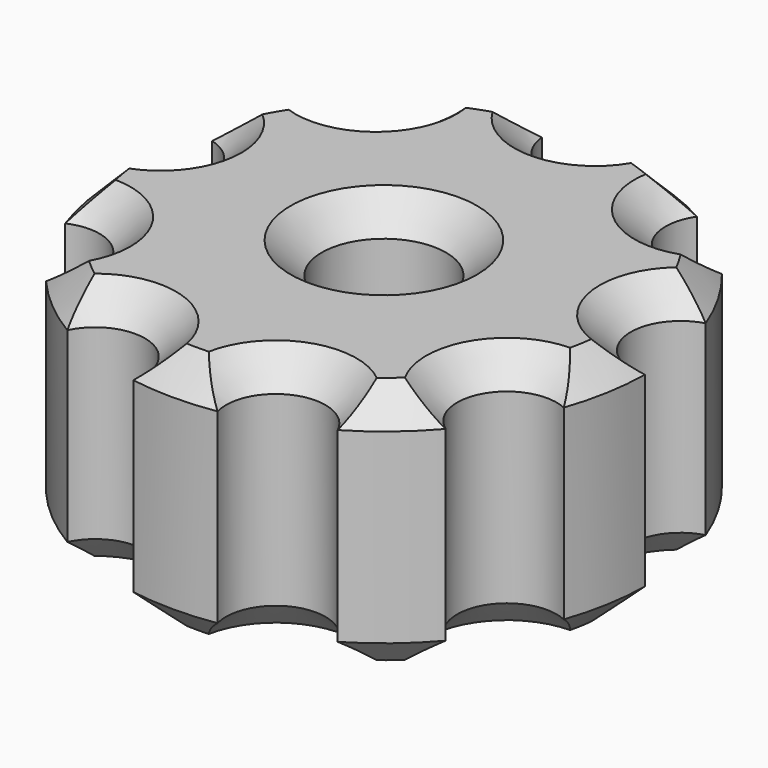
from build123d import *

# Parameters (mm, degrees)
F0_R         = 2
F1_DEPTH     = 8
F2_T2_ANGLE  = 353.6374425132
F2_T4_ANGLE  = 53.075870109
F2_T6_ANGLE  = 353.6374425132
F2_T8_ANGLE  = 53.075870109
F2_T10_ANGLE = 353.6374425132
F2_T12_ANGLE = 53.075870109
F2_T14_ANGLE = 353.6374425132
F2_T16_ANGLE = 53.075870109
F2_T18_ANGLE = 353.6374425132
F2_T20_ANGLE = 53.075870109
F2_T22_ANGLE = 353.6374425132
F2_T24_ANGLE = 53.075870109
F2_T26_ANGLE = 353.6374425132
F2_T28_ANGLE = 53.075870109
F2_T30_ANGLE = 353.6374425132
F2_T32_ANGLE = 53.075870109
F2_T34_ANGLE = 353.6374425132
F2_T36_ANGLE = 53.075870109
F2_T40_ANGLE = 353.6374425132
F2_T42_ANGLE = 53.075870109
F2_T44_ANGLE = 353.6374425132
F2_T46_ANGLE = 53.075870109
F2_T48_ANGLE = 353.6374425132
F2_T50_ANGLE = 53.075870109
F2_T52_ANGLE = 353.6374425132
F2_T54_ANGLE = 53.075870109
F2_T56_ANGLE = 353.6374425132
F2_T58_ANGLE = 53.075870109
F2_T60_ANGLE = 353.6374425132
F2_T62_ANGLE = 53.075870109
F2_T64_ANGLE = 353.6374425132
F2_T66_ANGLE = 53.075870109
F2_T68_ANGLE = 353.6374425132
F2_T70_ANGLE = 53.075870109
F2_T72_ANGLE = 353.6374425132
F2_T74_ANGLE = 53.075870109


# Not quite as in the source:
# - a fillet or chamfer that OpenCascade refuses, or shapes differently, is made with other operations: its cross-section is extruded or revolved along the edge and cut away or added


with BuildPart() as f1:
    # F0 (on Top) → F1 (new body)
    with BuildSketch(Plane.XY):
        with BuildLine():
            ThreePointArc((8.4941564461, -0.1197132759), (6.790249457, 1.197304185), (7.9409517805, 3.0176662871))
            ThreePointArc((7.9409517805, 3.0176662871), (7.3568858051, 4.2475), (6.583851555, 5.3682328285))
            ThreePointArc((6.583851555, 5.3682328285), (4.4320205688, 5.2818764353), (4.1434034849, 7.416011904))
            ThreePointArc((4.1434034849, 7.416011904), (2.9054611176, 7.9826888136), (1.59288935, 8.3443231313))
            ThreePointArc((1.59288935, 8.3443231313), (0, 6.895), (-1.59288935, 8.3443231313))
            ThreePointArc((-1.59288935, 8.3443231313), (-2.9054611176, 7.9826888136), (-4.1434034849, 7.416011904))
            ThreePointArc((-4.1434034849, 7.416011904), (-3.932847998, 6.983297681), (-3.8604807443, 6.5075475443))
            ThreePointArc((-3.8604807443, 6.5075475443), (-4.8429830913, 5.0315066747), (-6.583851555, 5.3682328285))
            ThreePointArc((-6.583851555, 5.3682328285), (-7.3568858051, 4.2475), (-7.9409517805, 3.0176662871))
            ThreePointArc((-7.9409517805, 3.0176662871), (-7.0931527728, 2.4446813329), (-6.7659418618, 1.4751412693))
            ThreePointArc((-6.7659418618, 1.4751412693), (-7.2808481642, 0.2993131919), (-8.4941564461, -0.1197132759))
            ThreePointArc((-8.4941564461, -0.1197132759), (-8.3659418618, -1.4751412693), (-8.022840484, -2.7926789231))
            ThreePointArc((-8.022840484, -2.7926789231), (-6.4924575219, -2.90111085), (-5.7568858051, -4.2475))
            ThreePointArc((-5.7568858051, -4.2475), (-5.9350743771, -4.9812930656), (-6.4299511341, -5.5516442081))
            ThreePointArc((-6.4299511341, -5.5516442081), (-5.4604807443, -6.5075475443), (-4.3507529612, -7.2962986281))
            ThreePointArc((-4.3507529612, -7.2962986281), (-2.5536564486, -6.4218449793), (-1.3054611176, -7.9826888136))
            ThreePointArc((-1.3054611176, -7.9826888136), (-1.318423401, -8.1859405941), (-1.3571002254, -8.3858991157))
            ThreePointArc((-1.3571002254, -8.3858991157), (0, -8.495), (1.3571002254, -8.3858991157))
            ThreePointArc((1.3571002254, -8.3858991157), (2.3582288882, -6.4791806203), (4.3507529612, -7.2962986281))
            ThreePointArc((4.3507529612, -7.2962986281), (5.4604807443, -6.5075475443), (6.4299511341, -5.5516442081))
            ThreePointArc((6.4299511341, -5.5516442081), (5.9712451591, -3.4475), (8.022840484, -2.7926789231))
            ThreePointArc((8.022840484, -2.7926789231), (8.3659418618, -1.4751412693), (8.4941564461, -0.1197132759))
        make_face()
        Circle(F0_R, mode=Mode.SUBTRACT)
    extrude(amount=F1_DEPTH)

    # F2: chamfer of 1 on 38 edges, made by hand

    # F2_s1 → F2_t2 (revolve, cut)
    with BuildSketch(Plane(origin=(0.2580100634, 0.3945620225, 0), x_dir=(0, 0, 1), z_dir=(0.5472897836, 0.8369431837, 0))):
        Polygon((7, 10.0819087839), (8, 11.0819087839), (8, 10.0819087839), align=None)
    revolve(axis=Axis((7.3568858051, -4.2475, 8), (0, 0, -1)), revolution_arc=F2_T2_ANGLE, mode=Mode.SUBTRACT)

    # F2_s3 → F2_t4 (revolve, cut)
    with BuildSketch(Plane(origin=(0, 0, 0), x_dir=(0, 0, 1), z_dir=(-0.5953548832, -0.8034628573, 0))):
        Polygon((8, -7.495), (7, -8.495), (8, -8.495), align=None)
    revolve(axis=Axis((0, 0, 8), (0, 0, 1)), revolution_arc=F2_T4_ANGLE, mode=Mode.SUBTRACT)

    # F2_s5 → F2_t6 (revolve, cut)
    with BuildSketch(Plane(origin=(-0.055972404, 0.4680977167, 0), x_dir=(0, 0, 1), z_dir=(-0.118728411, 0.9929267669, 0))):
        Polygon((8, 11.0819087839), (7, 10.0819087839), (8, 10.0819087839), align=None)
    revolve(axis=Axis((8.3659418618, 1.4751412693, 8), (0, 0, -1)), revolution_arc=F2_T6_ANGLE, mode=Mode.SUBTRACT)

    # F2_s7 → F2_t8 (revolve, cut)
    with BuildSketch(Plane(origin=(0, 0, 0), x_dir=(0, 0, 1), z_dir=(0.0603876695, -0.9981749994, 0))):
        Polygon((8, -7.495), (7, -8.495), (8, -8.495), align=None)
    revolve(axis=Axis((0, 0, 8), (0, 0, 1)), revolution_arc=F2_T8_ANGLE, mode=Mode.SUBTRACT)

    # F2_s9 → F2_t10 (revolve, cut)
    with BuildSketch(Plane(origin=(-0.3437647615, 0.322605287, 0), x_dir=(0, 0, 1), z_dir=(-0.7291922626, 0.6843088807, 0))):
        Polygon((8, 11.0819087839), (7, 10.0819087839), (8, 10.0819087839), align=None)
    revolve(axis=Axis((5.4604807443, 6.5075475443, 8), (0, 0, -1)), revolution_arc=F2_T10_ANGLE, mode=Mode.SUBTRACT)

    # F2_s11 → F2_t12 (revolve, cut)
    with BuildSketch(Plane(origin=(0, 0, 0), x_dir=(0, 0, 1), z_dir=(0.6878741606, -0.7258299658, 0))):
        Polygon((8, -7.495), (7, -8.495), (8, -8.495), align=None)
    revolve(axis=Axis((0, 0, 8), (0, 0, 1)), revolution_arc=F2_T12_ANGLE, mode=Mode.SUBTRACT)

    # F2_s13 → F2_t14 (revolve, cut)
    with BuildSketch(Plane(origin=(-0.4707057666, 0.0261622581, 0), x_dir=(0, 0, 1), z_dir=(-0.9984589504, 0.0554952639, 0))):
        Polygon((8, 11.0819087839), (7, 10.0819087839), (8, 10.0819087839), align=None)
    revolve(axis=Axis((0, 8.495, 8), (0, 0, -1)), revolution_arc=F2_T14_ANGLE, mode=Mode.SUBTRACT)

    # F2_s15 → F2_t16 (revolve, cut)
    with BuildSketch(Plane(origin=(0, 0, 0), x_dir=(0, 0, 1), z_dir=(0.993496687, -0.1138610245, 0))):
        Polygon((8, -7.495), (7, -8.495), (8, -8.495), align=None)
    revolve(axis=Axis((0, 0, 8), (0, 0, 1)), revolution_arc=F2_T16_ANGLE, mode=Mode.SUBTRACT)

    # F2_s17 → F2_t18 (revolve, cut)
    with BuildSketch(Plane(origin=(0.3437647615, 0.322605287, 0), x_dir=(0, 0, 1), z_dir=(0.7291922626, 0.6843088807, 0))):
        Polygon((8, -11.0819087839), (7, -10.0819087839), (8, -10.0819087839), align=None)
    revolve(axis=Axis((-5.4604807443, 6.5075475443, 8), (0, 0, 1)), revolution_arc=F2_T18_ANGLE, mode=Mode.SUBTRACT)

    # F2_s19 → F2_t20 (revolve, cut)
    with BuildSketch(Plane(origin=(0, 0, 0), x_dir=(0, 0, 1), z_dir=(0.8342510721, 0.5513847556, 0))):
        Polygon((8, -7.495), (7, -8.495), (8, -8.495), align=None)
    revolve(axis=Axis((0, 0, 8), (0, 0, 1)), revolution_arc=F2_T20_ANGLE, mode=Mode.SUBTRACT)

    # F2_s21 → F2_t22 (revolve, cut)
    with BuildSketch(Plane(origin=(0.055972404, 0.4680977167, 0), x_dir=(0, 0, 1), z_dir=(0.118728411, 0.9929267669, 0))):
        Polygon((8, -11.0819087839), (7, -10.0819087839), (8, -10.0819087839), align=None)
    revolve(axis=Axis((-8.3659418618, 1.4751412693, 8), (0, 0, 1)), revolution_arc=F2_T22_ANGLE, mode=Mode.SUBTRACT)

    # F2_s23 → F2_t24 (revolve, cut)
    with BuildSketch(Plane(origin=(0, 0, 0), x_dir=(0, 0, 1), z_dir=(0.2846501089, 0.9586314806, 0))):
        Polygon((8, -7.495), (7, -8.495), (8, -8.495), align=None)
    revolve(axis=Axis((0, 0, 8), (0, 0, 1)), revolution_arc=F2_T24_ANGLE, mode=Mode.SUBTRACT)

    # F2_s25 → F2_t26 (revolve, cut)
    with BuildSketch(Plane(origin=(-0.2580100634, 0.3945620225, 0), x_dir=(0, 0, 1), z_dir=(-0.5472897836, 0.8369431837, 0))):
        Polygon((8, -11.0819087839), (7, -10.0819087839), (8, -10.0819087839), align=None)
    revolve(axis=Axis((-7.3568858051, -4.2475, 8), (0, 0, 1)), revolution_arc=F2_T26_ANGLE, mode=Mode.SUBTRACT)

    # F2_s27 → F2_t28 (revolve, cut)
    with BuildSketch(Plane(origin=(0, 0, 0), x_dir=(0, 0, 1), z_dir=(-0.3981418038, 0.9173238818, 0))):
        Polygon((8, -7.495), (7, -8.495), (8, -8.495), align=None)
    revolve(axis=Axis((0, 0, 8), (0, 0, 1)), revolution_arc=F2_T28_ANGLE, mode=Mode.SUBTRACT)

    # F2_s29 → F2_t30 (revolve, cut)
    with BuildSketch(Plane(origin=(-0.4512667547, 0.1364063729, 0), x_dir=(0, 0, 1), z_dir=(-0.957225006, 0.2893445833, 0))):
        Polygon((8, -11.0819087839), (7, -10.0819087839), (8, -10.0819087839), align=None)
    revolve(axis=Axis((-2.9054611176, -7.9826888136, 8), (0, 0, 1)), revolution_arc=F2_T30_ANGLE, mode=Mode.SUBTRACT)

    # F2_s31 → F2_t32 (revolve, cut)
    with BuildSketch(Plane(origin=(0, 0, 0), x_dir=(0, 0, 1), z_dir=(-0.8946387416, 0.4467902438, 0))):
        Polygon((8, -7.495), (7, -8.495), (8, -8.495), align=None)
    revolve(axis=Axis((0, 0, 8), (0, 0, 1)), revolution_arc=F2_T32_ANGLE, mode=Mode.SUBTRACT)

    # F2_s33 → F2_t34 (revolve, cut)
    with BuildSketch(Plane(origin=(0.4512667547, 0.1364063729, 0), x_dir=(0, 0, 1), z_dir=(0.957225006, 0.2893445833, 0))):
        Polygon((8, 11.0819087839), (7, 10.0819087839), (8, 10.0819087839), align=None)
    revolve(axis=Axis((2.9054611176, -7.9826888136, 8), (0, 0, -1)), revolution_arc=F2_T34_ANGLE, mode=Mode.SUBTRACT)

    # F2_s35 → F2_t36 (revolve, cut)
    with BuildSketch(Plane(origin=(0, 0, 0), x_dir=(0, 0, 1), z_dir=(-0.9725242695, -0.2328015148, 0))):
        Polygon((8, -7.495), (7, -8.495), (8, -8.495), align=None)
    revolve(axis=Axis((0, 0, 8), (0, 0, 1)), revolution_arc=F2_T36_ANGLE, mode=Mode.SUBTRACT)

    # F2_s37 → F2_t38 (revolve, cut)
    with BuildSketch(Plane.XZ):
        Polygon((3, 8), (2, 7), (2, 8), align=None)
    revolve(axis=Axis((0, 0, 8), (0, 0, 1)), mode=Mode.SUBTRACT)

    # F2_s39 → F2_t40 (revolve, cut)
    with BuildSketch(Plane(origin=(0.2580100634, 0.3945620225, 0), x_dir=(0, 0, 1), z_dir=(0.5472897836, 0.8369431837, 0))):
        Polygon((1, 10.0819087839), (0, 11.0819087839), (0, 10.0819087839), align=None)
    revolve(axis=Axis((7.3568858051, -4.2475, 0), (0, 0, -1)), revolution_arc=F2_T40_ANGLE, mode=Mode.SUBTRACT)

    # F2_s41 → F2_t42 (revolve, cut)
    with BuildSketch(Plane(origin=(0, 0, 0), x_dir=(0, 0, 1), z_dir=(-0.5953548832, -0.8034628573, 0))):
        Polygon((0, -7.495), (1, -8.495), (0, -8.495), align=None)
    revolve(axis=Axis((0, 0, 0), (0, 0, 1)), revolution_arc=F2_T42_ANGLE, mode=Mode.SUBTRACT)

    # F2_s43 → F2_t44 (revolve, cut)
    with BuildSketch(Plane(origin=(-0.055972404, 0.4680977167, 0), x_dir=(0, 0, 1), z_dir=(-0.118728411, 0.9929267669, 0))):
        Polygon((1, 10.0819087839), (0, 11.0819087839), (0, 10.0819087839), align=None)
    revolve(axis=Axis((8.3659418618, 1.4751412693, 0), (0, 0, -1)), revolution_arc=F2_T44_ANGLE, mode=Mode.SUBTRACT)

    # F2_s45 → F2_t46 (revolve, cut)
    with BuildSketch(Plane(origin=(0, 0, 0), x_dir=(0, 0, 1), z_dir=(0.0603876695, -0.9981749994, 0))):
        Polygon((1, -8.495), (0, -7.495), (0, -8.495), align=None)
    revolve(axis=Axis((0, 0, 0), (0, 0, 1)), revolution_arc=F2_T46_ANGLE, mode=Mode.SUBTRACT)

    # F2_s47 → F2_t48 (revolve, cut)
    with BuildSketch(Plane(origin=(-0.3437647615, 0.322605287, 0), x_dir=(0, 0, 1), z_dir=(-0.7291922626, 0.6843088807, 0))):
        Polygon((1, 10.0819087839), (0, 11.0819087839), (0, 10.0819087839), align=None)
    revolve(axis=Axis((5.4604807443, 6.5075475443, 0), (0, 0, -1)), revolution_arc=F2_T48_ANGLE, mode=Mode.SUBTRACT)

    # F2_s49 → F2_t50 (revolve, cut)
    with BuildSketch(Plane(origin=(0, 0, 0), x_dir=(0, 0, 1), z_dir=(0.6878741606, -0.7258299658, 0))):
        Polygon((1, -8.495), (0, -7.495), (0, -8.495), align=None)
    revolve(axis=Axis((0, 0, 0), (0, 0, 1)), revolution_arc=F2_T50_ANGLE, mode=Mode.SUBTRACT)

    # F2_s51 → F2_t52 (revolve, cut)
    with BuildSketch(Plane(origin=(-0.4707057666, 0.0261622581, 0), x_dir=(0, 0, 1), z_dir=(-0.9984589504, 0.0554952639, 0))):
        Polygon((1, 10.0819087839), (0, 11.0819087839), (0, 10.0819087839), align=None)
    revolve(axis=Axis((0, 8.495, 0), (0, 0, -1)), revolution_arc=F2_T52_ANGLE, mode=Mode.SUBTRACT)

    # F2_s53 → F2_t54 (revolve, cut)
    with BuildSketch(Plane(origin=(0, 0, 0), x_dir=(0, 0, 1), z_dir=(0.993496687, -0.1138610245, 0))):
        Polygon((1, -8.495), (0, -7.495), (0, -8.495), align=None)
    revolve(axis=Axis((0, 0, 0), (0, 0, 1)), revolution_arc=F2_T54_ANGLE, mode=Mode.SUBTRACT)

    # F2_s55 → F2_t56 (revolve, cut)
    with BuildSketch(Plane(origin=(-0.3773983122, -0.2825223821, 0), x_dir=(0, 0, 1), z_dir=(-0.8005355987, -0.5992852036, 0))):
        Polygon((1, 10.0819087839), (0, 11.0819087839), (0, 10.0819087839), align=None)
    revolve(axis=Axis((-5.4604807443, 6.5075475443, 0), (0, 0, -1)), revolution_arc=F2_T56_ANGLE, mode=Mode.SUBTRACT)

    # F2_s57 → F2_t58 (revolve, cut)
    with BuildSketch(Plane(origin=(0, 0, 0), x_dir=(0, 0, 1), z_dir=(0.8342510721, 0.5513847556, 0))):
        Polygon((1, -8.495), (0, -7.495), (0, -8.495), align=None)
    revolve(axis=Axis((0, 0, 0), (0, 0, 1)), revolution_arc=F2_T58_ANGLE, mode=Mode.SUBTRACT)

    # F2_s59 → F2_t60 (revolve, cut)
    with BuildSketch(Plane(origin=(-0.1075019932, -0.4590116599, 0), x_dir=(0, 0, 1), z_dir=(-0.2280327434, -0.973653464, 0))):
        Polygon((1, 10.0819087839), (0, 11.0819087839), (0, 10.0819087839), align=None)
    revolve(axis=Axis((-8.3659418618, 1.4751412693, 0), (0, 0, -1)), revolution_arc=F2_T60_ANGLE, mode=Mode.SUBTRACT)

    # F2_s61 → F2_t62 (revolve, cut)
    with BuildSketch(Plane(origin=(0, 0, 0), x_dir=(0, 0, 1), z_dir=(0.2846501089, 0.9586314806, 0))):
        Polygon((1, -8.495), (0, -7.495), (0, -8.495), align=None)
    revolve(axis=Axis((0, 0, 0), (0, 0, 1)), revolution_arc=F2_T62_ANGLE, mode=Mode.SUBTRACT)

    # F2_s63 → F2_t64 (revolve, cut)
    with BuildSketch(Plane(origin=(0.2126957032, -0.4207242806, 0), x_dir=(0, 0, 1), z_dir=(0.4511691669, -0.8924384477, 0))):
        Polygon((1, 10.0819087839), (0, 11.0819087839), (0, 10.0819087839), align=None)
    revolve(axis=Axis((-7.3568858051, -4.2475, 0), (0, 0, -1)), revolution_arc=F2_T64_ANGLE, mode=Mode.SUBTRACT)

    # F2_s65 → F2_t66 (revolve, cut)
    with BuildSketch(Plane(origin=(0, 0, 0), x_dir=(0, 0, 1), z_dir=(-0.3981418038, 0.9173238818, 0))):
        Polygon((1, -8.495), (0, -7.495), (0, -8.495), align=None)
    revolve(axis=Axis((0, 0, 0), (0, 0, 1)), revolution_arc=F2_T66_ANGLE, mode=Mode.SUBTRACT)

    # F2_s67 → F2_t68 (revolve, cut)
    with BuildSketch(Plane(origin=(0.4333707161, -0.1855753346, 0), x_dir=(0, 0, 1), z_dir=(0.9192640097, -0.3936415633, 0))):
        Polygon((1, 10.0819087839), (0, 11.0819087839), (0, 10.0819087839), align=None)
    revolve(axis=Axis((-2.9054611176, -7.9826888136, 0), (0, 0, -1)), revolution_arc=F2_T68_ANGLE, mode=Mode.SUBTRACT)

    # F2_s69 → F2_t70 (revolve, cut)
    with BuildSketch(Plane(origin=(0, 0, 0), x_dir=(0, 0, 1), z_dir=(-0.8946387416, 0.4467902438, 0))):
        Polygon((1, -8.495), (0, -7.495), (0, -8.495), align=None)
    revolve(axis=Axis((0, 0, 0), (0, 0, 1)), revolution_arc=F2_T70_ANGLE, mode=Mode.SUBTRACT)

    # F2_s71 → F2_t72 (revolve, cut)
    with BuildSketch(Plane(origin=(0.4512667547, 0.1364063729, 0), x_dir=(0, 0, 1), z_dir=(0.957225006, 0.2893445833, 0))):
        Polygon((1, 10.0819087839), (0, 11.0819087839), (0, 10.0819087839), align=None)
    revolve(axis=Axis((2.9054611176, -7.9826888136, 0), (0, 0, -1)), revolution_arc=F2_T72_ANGLE, mode=Mode.SUBTRACT)

    # F2_s73 → F2_t74 (revolve, cut)
    with BuildSketch(Plane(origin=(0, 0, 0), x_dir=(0, 0, 1), z_dir=(-0.9725242695, -0.2328015148, 0))):
        Polygon((0, -7.495), (1, -8.495), (0, -8.495), align=None)
    revolve(axis=Axis((0, 0, 0), (0, 0, 1)), revolution_arc=F2_T74_ANGLE, mode=Mode.SUBTRACT)

    # F2_s75 → F2_t76 (revolve, cut)
    with BuildSketch(Plane.XZ):
        Polygon((2, 1), (3, 0), (2, 0), align=None)
    revolve(axis=Axis((0, 0, 0), (0, 0, 1)), mode=Mode.SUBTRACT)


solid = f1.part
